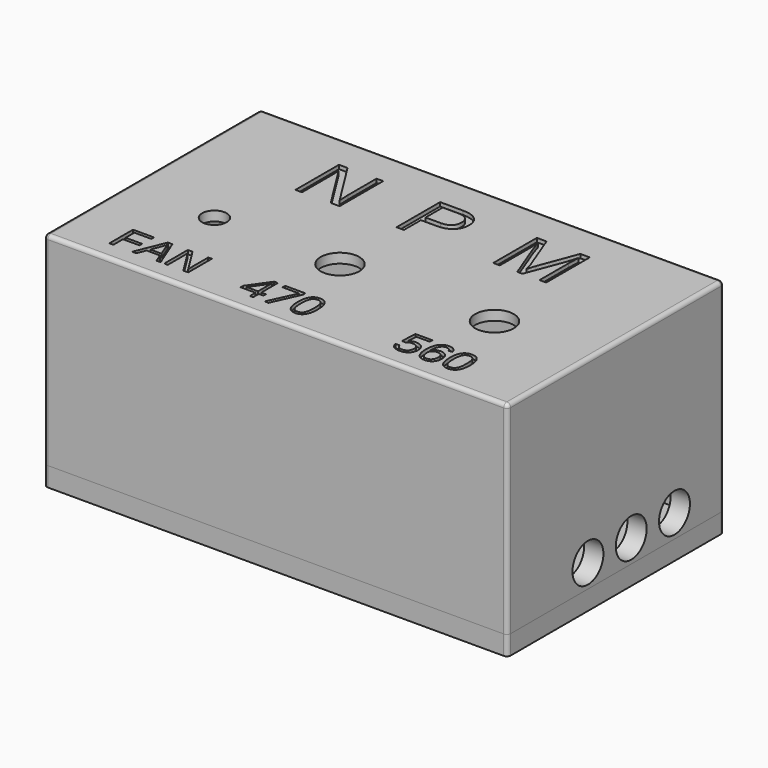
from build123d import *

# Parameters (mm, degrees)
F0_W             = 120
F0_H             = 70
F0_R             = 3.175
F0_R_2           = 5
F1_DEPTH         = 2.5
F2_W             = 120
F2_H             = 70
F2_W_2           = 110
F2_H_2           = 60
F3_DEPTH         = 50
F4_W             = 120
F4_H             = 70
F4_W_2           = 110
F4_H_2           = 60
F5_DEPTH         = 5
F7_D             = 2.4
F7_DEPTH         = 5
F7_CSINK_D       = 4
F7_CSINK_ANGLE   = 90
F7_TIP           = 0.7210327428
F7_2_D           = 2.4
F7_2_DEPTH       = 5
F7_2_CSINK_D     = 4
F7_2_CSINK_ANGLE = 90
F7_2_TIP         = 0.7210327428
F9_D             = 2.9
F9_DEPTH         = 5.2
F9_CBORE_D       = 3.7
F9_CBORE_DEPTH   = 0.2
F9_TIP           = 0.8712478976
F10_R            = 1
F10_2_R          = 1
F11_R            = 5
F12_DEPTH        = 5
F13_R            = 5
F14_DEPTH        = 5
F15_TEXT_SIZE    = 20.4861111111
F16_DEPTH        = 1
F17_TEXT_SIZE    = 11.1111111111
F18_DEPTH        = 1
F20_D            = 6.3
F20_DEPTH        = 5.2
F20_CSINK_D      = 12.1
F20_CSINK_ANGLE  = 90
F20_TIP          = 1.8927109499


# Not quite as in the source:
# - Text() gives the source's letters only with a copy of the font that has no kerning and outlines rounded to 1/6400 em; it was checked with that copy


with BuildPart() as f1:
    # F0 (on Top) → F1 (new body)
    with BuildSketch(Plane.XY):
        with Locations((60, 35)):
            Rectangle(F0_W, F0_H)
        with Locations((22.5, 27)):
            Circle(F0_R, mode=Mode.SUBTRACT)
        with Locations((55, 27)):
            Circle(F0_R_2, mode=Mode.SUBTRACT)
        with Locations((95, 27)):
            Circle(F0_R_2, mode=Mode.SUBTRACT)
    extrude(amount=F1_DEPTH)

    # F2 (on face) → F3 (join)
    with BuildSketch(Plane(origin=(0, 0, 0), x_dir=(1, 0, 0), z_dir=(0, 0, -1))):
        with Locations((60, -35)):
            Rectangle(F2_W, F2_H)
        with Locations((60, -35)):
            Rectangle(F2_W_2, F2_H_2, mode=Mode.SUBTRACT)
    extrude(amount=F3_DEPTH)

    # F7
    with Locations(Plane(origin=(0, 0, -55), x_dir=(1, 0, 0), z_dir=(0, 0, -1))):
        with Locations((2.5, -2.5), (2.5, -67.5), (117.5, -67.5), (117.5, -2.5)):
            CounterSinkHole(F7_D / 2, F7_CSINK_D / 2, depth=F7_DEPTH, counter_sink_angle=F7_CSINK_ANGLE)
            with Locations((0, 0, -(F7_DEPTH + F7_TIP / 2))):  # 118° drill point
                Cone(0, F7_D / 2, F7_TIP, mode=Mode.SUBTRACT)

    # F9
    with Locations(Plane(origin=(0, 0, -50), x_dir=(1, 0, 0), z_dir=(0, 0, -1))):
        with Locations((2.5, -2.5), (2.5, -67.5), (117.5, -67.5), (117.5, -2.5)):
            CounterBoreHole(F9_D / 2, F9_CBORE_D / 2, F9_CBORE_DEPTH, depth=F9_DEPTH)
            with Locations((0, 0, -(F9_DEPTH + F9_TIP / 2))):  # 118° drill point
                Cone(0, F9_D / 2, F9_TIP, mode=Mode.SUBTRACT)

    # F10
    f10_edges = [f1.edges().sort_by_distance(p)[0] for p in [
        (60, 0, 2.5),
        (0, 35, 2.5),
        (60, 70, 2.5),
        (120, 35, 2.5),
        (120, 0, -23.75),
        (0, 0, -23.75),
        (120, 70, -23.75),
        (0, 70, -23.75),
    ]]
    fillet(f10_edges, radius=F10_R)

    # F11 (on face) → F12 (cut, through all)
    with BuildSketch(Plane(origin=(0, 0, 0), x_dir=(0, -1, 0), z_dir=(-1, 0, 0))):
        with Locations((-18, -44)):
            Circle(F11_R)
    extrude(amount=-F12_DEPTH, mode=Mode.SUBTRACT)

    # F13 (on face) → F14 (cut, through all)
    with BuildSketch(Plane.YZ.offset(120)):
        with Locations((26, -44)):
            Circle(F13_R)
        with Locations((40, -44)):
            Circle(F13_R)
        with Locations((54, -44)):
            Circle(F13_R)
    extrude(amount=-F14_DEPTH, mode=Mode.SUBTRACT)

    # F15 (on face) → F16 (cut)
    with BuildSketch(Plane.XY.offset(2.5)):
        with Locations((25.9850531684, 46.75)):
            Text('N  P  M', F15_TEXT_SIZE, font='Arimo', text_align=(TextAlign.LEFT, TextAlign.BOTTOM))
    extrude(amount=-F16_DEPTH, mode=Mode.SUBTRACT)

    # F17 (on face) → F18 (cut)
    with BuildSketch(Plane.XY.offset(2.5)):
        with Locations((12, 5)):
            Text('FAN', F17_TEXT_SIZE, font='Arimo', text_align=(TextAlign.LEFT, TextAlign.BOTTOM))
        with Locations((85.1267361111, 5)):
            Text('560', F17_TEXT_SIZE, font='Arimo', text_align=(TextAlign.LEFT, TextAlign.BOTTOM))
        with Locations((45.4010416667, 4.7221066505)):
            Text('470', F17_TEXT_SIZE, font='Open Sans', text_align=(TextAlign.LEFT, TextAlign.BOTTOM))
    extrude(amount=-F18_DEPTH, mode=Mode.SUBTRACT)


with BuildPart() as f5:
    # F4 (on face) → F5 (new body)
    with BuildSketch(Plane(origin=(0, 0, -50), x_dir=(1, 0, 0), z_dir=(0, 0, -1))):
        with Locations((60, -35)):
            Rectangle(F4_W, F4_H)
        with Locations((60, -35)):
            Rectangle(F4_W_2, F4_H_2, mode=Mode.SUBTRACT)
        with Locations((60, -35)):
            Rectangle(F4_W_2, F4_H_2)
    extrude(amount=F5_DEPTH)

    # F7#2
    with Locations(Plane(origin=(0, 0, -55), x_dir=(1, 0, 0), z_dir=(0, 0, -1))):
        with Locations((2.5, -2.5), (2.5, -67.5), (117.5, -67.5), (117.5, -2.5)):
            CounterSinkHole(F7_2_D / 2, F7_2_CSINK_D / 2, depth=F7_2_DEPTH, counter_sink_angle=F7_2_CSINK_ANGLE)
            with Locations((0, 0, -(F7_2_DEPTH + F7_2_TIP / 2))):  # 118° drill point
                Cone(0, F7_2_D / 2, F7_2_TIP, mode=Mode.SUBTRACT)

    # F10#2
    f10_2_edges = [f5.edges().sort_by_distance(p)[0] for p in [
        (0, 70, -52.5),
        (0, 0, -52.5),
        (120, 70, -52.5),
        (120, 0, -52.5),
    ]]
    fillet(f10_2_edges, radius=F10_2_R)

    # F20
    with Locations(Plane.XY.offset(-50)):
        with Locations((40, 35), (80, 35)):
            CounterSinkHole(F20_D / 2, F20_CSINK_D / 2, depth=F20_DEPTH, counter_sink_angle=F20_CSINK_ANGLE)
            with Locations((0, 0, -(F20_DEPTH + F20_TIP / 2))):  # 118° drill point
                Cone(0, F20_D / 2, F20_TIP, mode=Mode.SUBTRACT)


solid = Compound([f1.part, f5.part])
